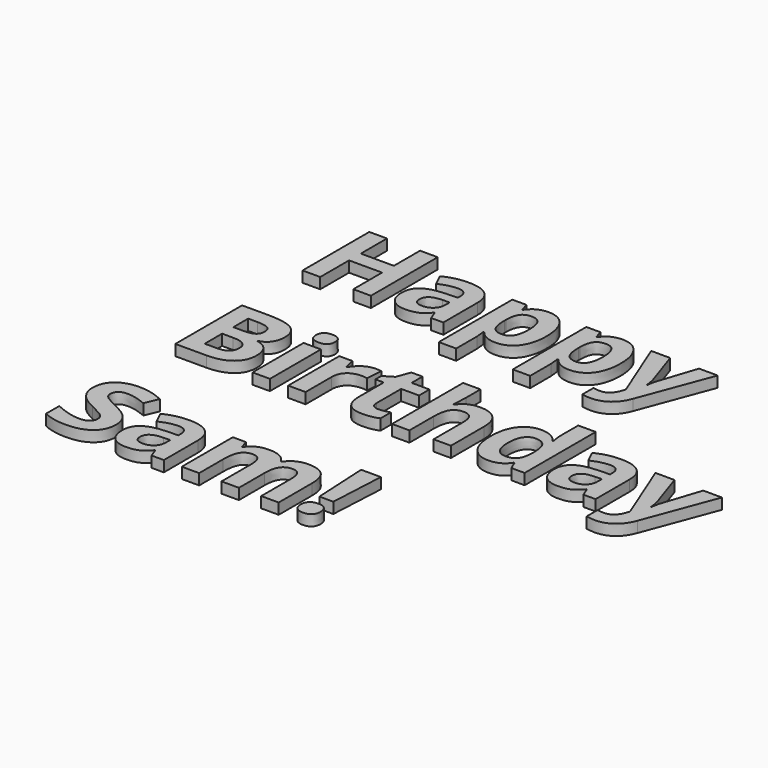
from build123d import *

# Parameters (mm, degrees)
F0_TEXT_SIZE = 53.8569719841
F1_DEPTH     = 5


# Not quite as in the source:
# - Text() gives the source's letters only with a copy of the font that has no kerning and outlines rounded to 1/6400 em; it was checked with that copy


with BuildPart() as f1:
    # F0 (on Top) → F1 (new body)
    with BuildSketch(Plane.XY):
        with Locations((0, 0)):
            Text('Happy', F0_TEXT_SIZE, font='Open Sans', font_style=FontStyle.BOLD, text_align=(TextAlign.LEFT, TextAlign.BOTTOM))
        with Locations((0, -73.2454818984)):
            Text('Birthday', F0_TEXT_SIZE, font='Open Sans', font_style=FontStyle.BOLD, text_align=(TextAlign.LEFT, TextAlign.BOTTOM))
        with Locations((0, -146.4909637968)):
            Text('Sam!', F0_TEXT_SIZE, font='Open Sans', font_style=FontStyle.BOLD, text_align=(TextAlign.LEFT, TextAlign.BOTTOM))
    extrude(amount=F1_DEPTH)


solid = f1.part
